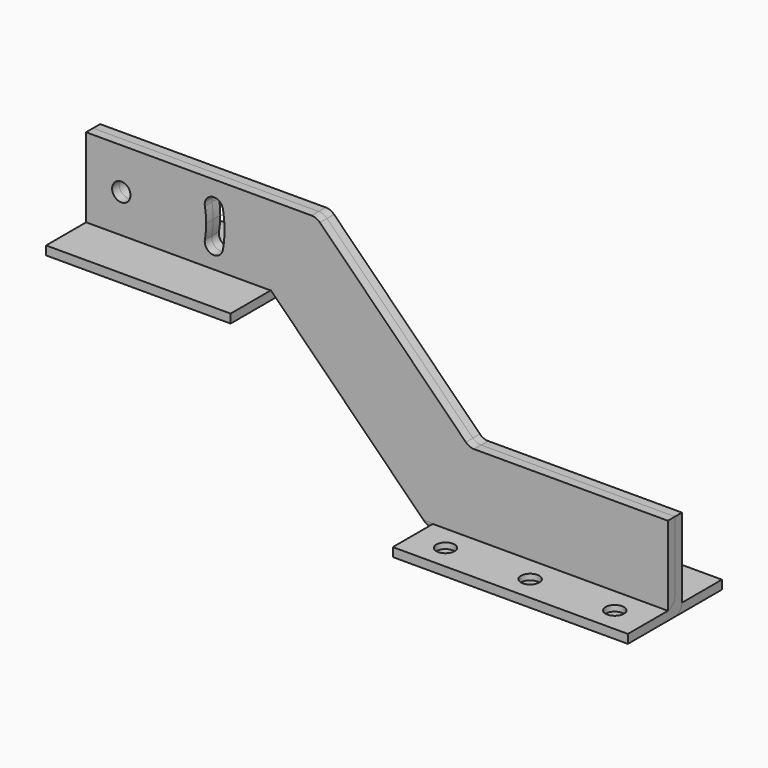
from build123d import *

# Parameters (mm, degrees)
F0_R        = 4.96062
F1_DEPTH    = 4.7625
F2_W        = 31.75
F2_H        = 4.7625
F3_DEPTH    = 127
F4_T1_DEPTH = 127
F4_T3_DEPTH = 152.4
F5_R        = 4.96062
F6_DEPTH    = 3.175
F7_W        = 31.75
F7_H        = 4.7625
F8_DEPTH    = 99.695
F9_R        = 5.08
F11_DEPTH   = 25.4


# Not quite as in the source:
# - a fillet or chamfer that OpenCascade refuses, or shapes differently, is made with other operations: its cross-section is extruded or revolved along the edge and cut away or added


with BuildPart() as f1:
    # F0 (on Front) → F1 (new body)
    with BuildSketch(Plane.XZ):
        with BuildLine():
            Line((-82.55, 82.55), (0, 0))
            Line((0, 0), (127, 0))
            Line((127, 0), (127, 47.625))
            Line((127, 47.625), (22.3571770291, 47.625))
            ThreePointArc((22.3571770291, 47.625), (19.9271372336, 48.1083649686), (17.8670489686, 49.4848719395))
            Line((17.8670489686, 49.4848719395), (-60.9632071525, 128.3151280605))
            ThreePointArc((-60.9632071525, 128.3151280605), (-63.0232954175, 129.6916350314), (-65.4533352131, 130.175))
            Line((-65.4533352131, 130.175), (-187.325, 130.175))
            Line((-187.325, 130.175), (-187.325, 82.55))
            Line((-187.325, 82.55), (-82.55, 82.55))
        make_face()
        with Locations((-168.275, 107.95)):
            Circle(F0_R, mode=Mode.SUBTRACT)
        with BuildLine():
            ThreePointArc((-113.3757178125, 117.6693530802), (-112.7358395418, 112.8283875), (-112.522, 107.95))
            ThreePointArc((-112.522, 107.95), (-112.7358395418, 103.0716125), (-113.3757178125, 98.2306469198))
            ThreePointArc((-113.3757178125, 98.2306469198), (-119.1163255014, 94.2169402337), (-123.1300321875, 99.9575479227))
            ThreePointArc((-123.1300321875, 99.9575479227), (-122.6038452724, 103.9383875), (-122.428, 107.95))
            ThreePointArc((-122.428, 107.95), (-122.6038452724, 111.9616125), (-123.1300321875, 115.9424520773))
            ThreePointArc((-123.1300321875, 115.9424520773), (-119.1163255014, 121.6830597663), (-113.3757178125, 117.6693530802))
        make_face(mode=Mode.SUBTRACT)
    extrude(amount=F1_DEPTH)

    # F2 (on face) → F3 (join)
    with BuildSketch(Plane.YZ.offset(127)):
        with Locations((15.875, 2.38125)):
            Rectangle(F2_W, F2_H)
    extrude(amount=-F3_DEPTH)

    # F4: fillet of radius 5.08 on 2 edges, made by hand

    # F4_s2 → F4_t1 (join)
    with BuildSketch(Plane.YZ):
        with BuildLine():
            ThreePointArc((5.08, 4.7625), (1.4878975516, 6.2503975516), (0, 9.8425))
            Line((0, 9.8425), (0, 4.7625))
            Line((0, 4.7625), (5.08, 4.7625))
        make_face()
    extrude(amount=F4_T1_DEPTH)

    # F4_s4 → F4_t3 (cut)
    with BuildSketch(Plane.YZ.offset(-12.7)):
        with BuildLine():
            ThreePointArc((-4.7625, 5.08), (-3.2746024484, 1.4878975516), (0.3175, 0))
            Line((0.3175, 0), (-4.7625, 0))
            Line((-4.7625, 0), (-4.7625, 5.08))
        make_face()
    extrude(amount=F4_T3_DEPTH, mode=Mode.SUBTRACT)

    # F5 (on face) → F6 (cut)
    with BuildSketch(Plane.XY.offset(4.7625)):
        with Locations((17.79778, 18.42008)):
            Circle(F5_R)
        with Locations((63.51778, 18.42008)):
            Circle(F5_R)
        with Locations((109.23778, 18.42008)):
            Circle(F5_R)
    extrude(amount=-F6_DEPTH, mode=Mode.SUBTRACT)

    # F7 (on face) → F8 (join)
    with BuildSketch(Plane(origin=(-187.325, 0, 0), x_dir=(0, -1, 0), z_dir=(-1, 0, 0))):
        with Locations((-15.875, 84.93125)):
            Rectangle(F7_W, F7_H)
    extrude(amount=-F8_DEPTH)

    # F9
    f9_edges = [f1.edges().sort_by_distance(p)[0] for p in [
        (-134.9375, -4.7625, 82.55),
        (-137.4775, 0, 87.3125),
    ]]
    fillet(f9_edges, radius=F9_R)

    # F10 (on face) → F11 (cut)
    with BuildSketch(Plane.XZ.offset(4.7625)):
        Polygon((-82.5599315833, 82.5599315833), (-87.63, 87.63), (-87.63, 82.5599315833), align=None)
    extrude(amount=-F11_DEPTH, mode=Mode.SUBTRACT)


with BuildPart() as f12_1:
    # F12: instance of F1
    add(f1.part.mirror(Plane.XZ))


solid = Compound([f1.part, f12_1.part])
